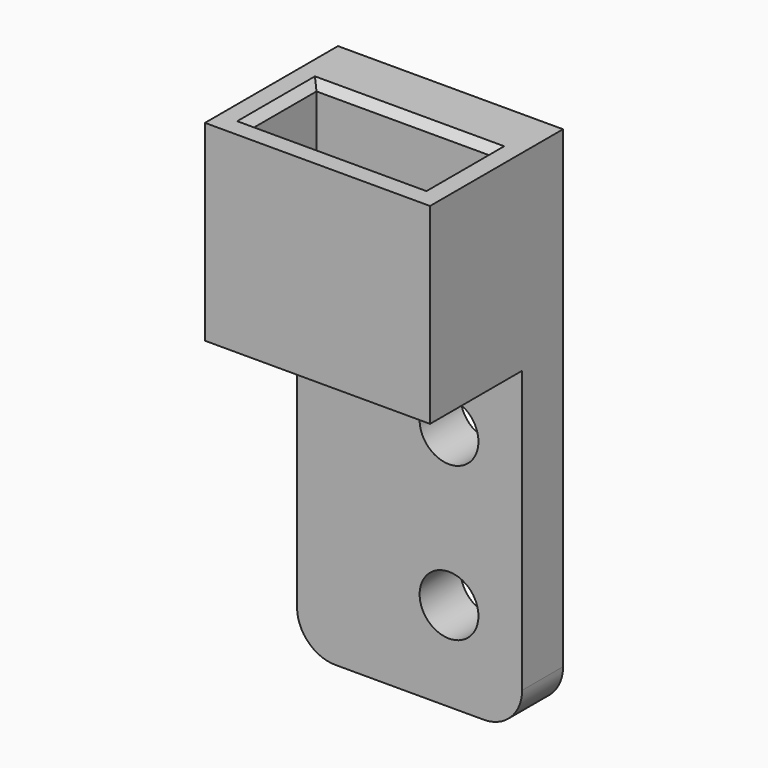
from build123d import *

# Parameters (mm, degrees)
F0_W     = 17.6
F0_H     = 9
F0_W_2   = 13.6
F0_H_2   = 6.4
F1_DEPTH = 7.5
F2_W     = 17.6
F2_H     = 15
F2_H_2   = 25
F3_DEPTH = 4
F4_SIZE  = 0.6
F5_D     = 4.6
F5_DEPTH = 10
F5_TIP   = 1.3819794238
F6_R     = 3


# Not quite as in the source:
# - a feature names something its author has since deleted; it is built from what else it names


with BuildPart() as f1:
    # F0 (on Top) → F1 (new body, symmetric)
    with BuildSketch(Plane.XY):
        with Locations((-5.2887722373, 2.4212898893)):
            Rectangle(F0_W, F0_H)
        with Locations((-5.2887722373, 3.1212898893)):
            Rectangle(F0_W_2, F0_H_2, mode=Mode.SUBTRACT)
    extrude(amount=F1_DEPTH, both=True)

    # F2 (on face) → F3 (join)
    with BuildSketch(Plane(origin=(0, 6.9212898893, 0), x_dir=(-1, 0, 0), z_dir=(0, 1, 0))):
        with Locations((5.2887722373, 0)):
            Rectangle(F2_W, F2_H)
        with Locations((5.2887722373, -20)):
            Rectangle(F2_W, F2_H_2)
    extrude(amount=F3_DEPTH)

    # F4
    f4_edges = [f1.edges().sort_by_distance(p)[0] for p in [
        (-5.288772, 6.32129, 7.5),
        (1.511228, 3.12129, 7.5),
        (-12.088772, 3.12129, 7.5),
        (-5.288772, -0.07871, 7.5),
    ]]
    chamfer(f4_edges, length=F4_SIZE)

    # F5
    with Locations(Plane(origin=(0, 6.9212898893, 0), x_dir=(-1, 0, 0), z_dir=(0, -1, 0))):
        with Locations((2.2041960619, 25.4963655025), (2.2041960619, 13.4963655025)):
            Hole(F5_D / 2, depth=F5_DEPTH)
            with Locations((0, 0, -(F5_DEPTH + F5_TIP / 2))):  # 118° drill point
                Cone(0, F5_D / 2, F5_TIP, mode=Mode.SUBTRACT)

    # F6
    f6_edges = [f1.edges().sort_by_distance(p)[0] for p in [
        (3.511228, 8.92129, -32.5),
        (-14.088772, 8.92129, -32.5),
    ]]
    fillet(f6_edges, radius=F6_R)


solid = f1.part
